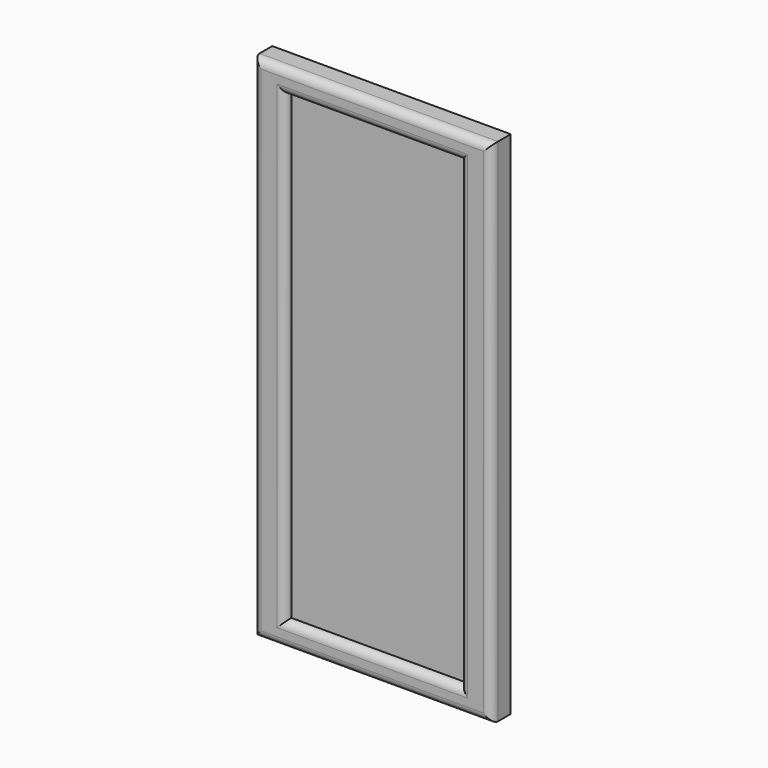
from build123d import *

# Parameters (mm, degrees)
F0_W     = 379.73
F0_H     = 812.8
F1_DEPTH = 25.4
F2_W     = 379.73
F2_H     = 812.8
F2_W_2   = 278.13
F2_H_2   = 736.6
F3_DEPTH = 12.7
F4_R     = 12.69999


# Not quite as in the source:
# - a fillet or chamfer is up to 0.001 mm smaller than in the source, because OpenCascade refuses the exact size


with BuildPart() as f1:
    # F0 (on Front) → F1 (new body)
    with BuildSketch(Plane.XZ):
        Rectangle(F0_W, F0_H)
    extrude(amount=F1_DEPTH)

    # F2 (on face) → F3 (join)
    with BuildSketch(Plane.XZ.offset(25.4)):
        Rectangle(F2_W, F2_H)
        Rectangle(F2_W_2, F2_H_2, mode=Mode.SUBTRACT)
    extrude(amount=F3_DEPTH)

    # F4 (radius 12.7 in the source; OpenCascade refuses exactly that, so slightly less here)
    f4_edges = [f1.edges().sort_by_distance(p)[0] for p in [
        (-189.865, -38.1, 0),
        (0, -38.1, -406.4),
        (189.865, -38.1, 0),
        (0, -38.1, 406.4),
        (-139.065, -38.1, 0),
        (0, -38.1, -368.3),
        (139.065, -38.1, 0),
        (0, -38.1, 368.3),
    ]]
    fillet(f4_edges, radius=F4_R)


solid = f1.part
